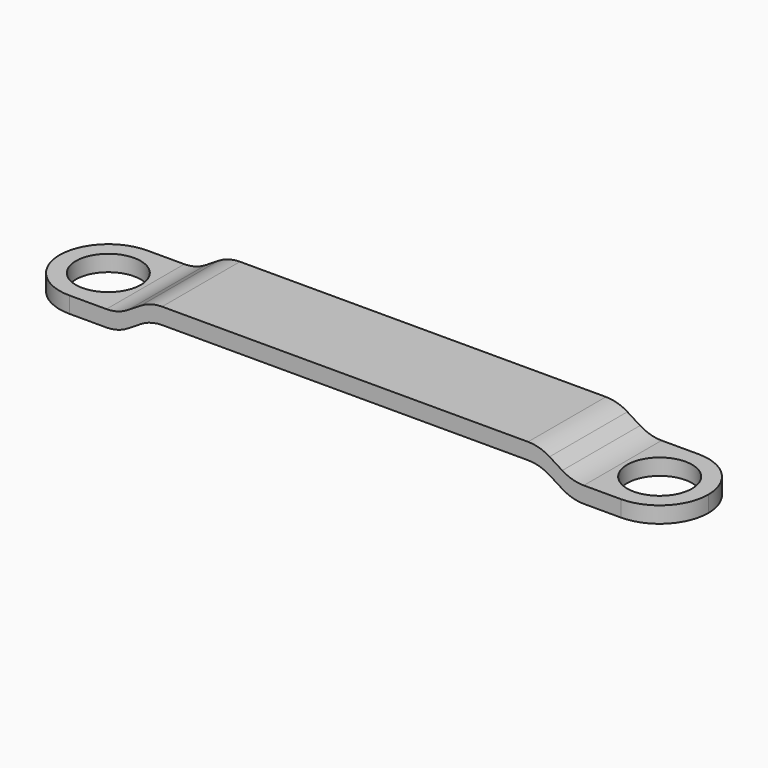
from build123d import *

# Parameters (mm, degrees)
F2_DEPTH = 3.81
F3_D     = 5.08
F3_DEPTH = 3.81
F3_TIP   = 1.5261859723
F4_R     = 3.80999


# Not quite as in the source:
# - a fillet or chamfer is up to 0.001 mm smaller than in the source, because OpenCascade refuses the exact size


with BuildPart() as f2:
    # F1 (on Front) → F2 (new body, symmetric)
    with BuildSketch(Plane.XZ):
        with BuildLine():
            Line((-25.4, 1.27), (-25.4, 0))
            Line((-25.4, 0), (-18.6905780189, 0))
            ThreePointArc((-18.6905780189, 0), (-17.8152860399, 0.1230352309), (-17.0078313843, 0.4826053848))
            Line((-17.0078313843, 0.4826053848), (-16.0121686157, 1.1048946152))
            ThreePointArc((-16.0121686157, 1.1048946152), (-15.2047139601, 1.4644647691), (-14.3294219811, 1.5875))
            Line((-14.3294219811, 1.5875), (14.3294219811, 1.5875))
            ThreePointArc((14.3294219811, 1.5875), (15.2047139601, 1.4644647691), (16.0121686157, 1.1048946152))
            Line((16.0121686157, 1.1048946152), (17.0078313843, 0.4826053848))
            ThreePointArc((17.0078313843, 0.4826053848), (17.8152860399, 0.1230352309), (18.6905780189, 0))
            Line((18.6905780189, 0), (25.4, 0))
            Line((25.4, 0), (25.4, 1.27))
            Line((25.4, 1.27), (18.6905780189, 1.27))
            ThreePointArc((18.6905780189, 1.27), (17.8152860399, 1.3930352309), (17.0078313843, 1.7526053848))
            Line((17.0078313843, 1.7526053848), (16.0121686157, 2.3748946152))
            ThreePointArc((16.0121686157, 2.3748946152), (15.2047139601, 2.7344647691), (14.3294219811, 2.8575))
            Line((14.3294219811, 2.8575), (-14.3294219811, 2.8575))
            ThreePointArc((-14.3294219811, 2.8575), (-15.2047139601, 2.7344647691), (-16.0121686157, 2.3748946152))
            Line((-16.0121686157, 2.3748946152), (-17.0078313843, 1.7526053848))
            ThreePointArc((-17.0078313843, 1.7526053848), (-17.8152860399, 1.3930352309), (-18.6905780189, 1.27))
            Line((-18.6905780189, 1.27), (-25.4, 1.27))
        make_face()
    extrude(amount=F2_DEPTH, both=True)

    # F3
    with Locations(Plane(origin=(0, 0, 0), x_dir=(1, 0, 0), z_dir=(0, 0, -1))):
        with Locations((-21.59, 0), (21.59, 0)):
            Hole(F3_D / 2, depth=F3_DEPTH)
            with Locations((0, 0, -(F3_DEPTH + F3_TIP / 2))):  # 118° drill point
                Cone(0, F3_D / 2, F3_TIP, mode=Mode.SUBTRACT)

    # F4 (radius 3.81 in the source; OpenCascade refuses exactly that, so slightly less here)
    f4_edges = [f2.edges().sort_by_distance(p)[0] for p in [
        (-25.4, -3.81, 0.635),
        (-25.4, 3.81, 0.635),
        (25.4, -3.81, 0.635),
        (25.4, 3.81, 0.635),
    ]]
    fillet(f4_edges, radius=F4_R)


solid = f2.part
